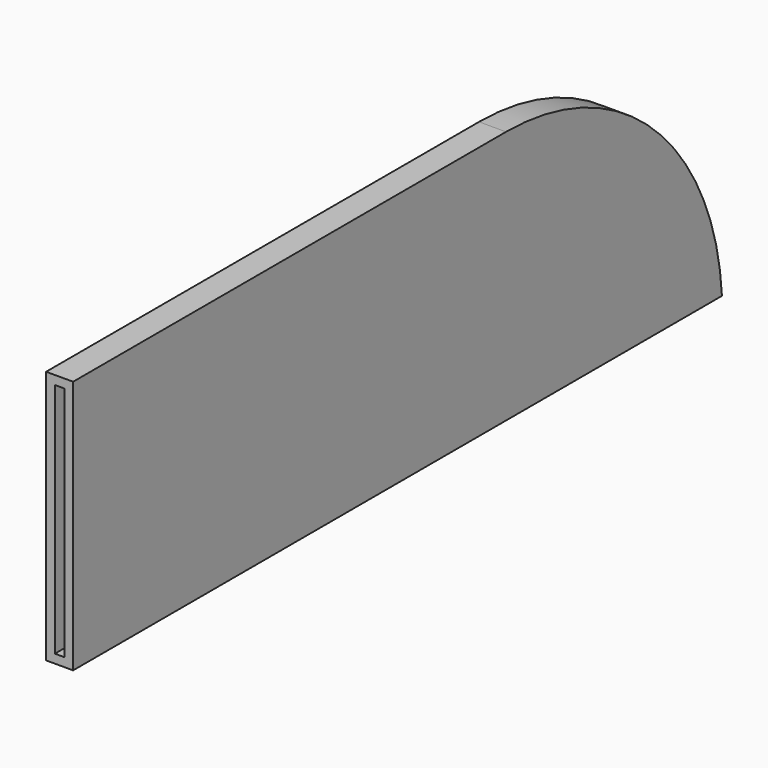
from build123d import *

# Parameters (mm, degrees)
F0_W        = 150
F0_H        = 47
F1_DEPTH    = 5
F2_T1_DEPTH = 254.5495942694
F3_T        = -1.625


# Not quite as in the source:
# - a fillet or chamfer that OpenCascade refuses, or shapes differently, is made with other operations: its cross-section is extruded or revolved along the edge and cut away or added


with BuildPart() as f1:
    # F0 (on Right) → F1 (new body)
    with BuildSketch(Plane.YZ):
        with Locations((9.6287353195, 42.6455706358)):
            Rectangle(F0_W, F0_H)
    extrude(amount=F1_DEPTH)

    # F2: fillet of radius 50 on 1 edges, made by hand

    # F2_s2 → F2_t1 (cut)
    with BuildSketch(Plane.YZ.offset(-124.7747971347)):
        with BuildLine():
            ThreePointArc((84.6287353195, 19.1455706358), (68.9970894677, 52.5461200822), (34.7188164657, 66.1455706358))
            Line((34.7188164657, 66.1455706358), (84.6287353195, 66.1455706358))
            Line((84.6287353195, 66.1455706358), (84.6287353195, 19.1455706358))
        make_face()
    extrude(amount=F2_T1_DEPTH, mode=Mode.SUBTRACT)

    # F3
    f3_openings = [f1.faces().sort_by_distance(p)[0] for p in [
        (2.5, -65.371265, 42.645571),
    ]]
    offset(amount=F3_T, openings=f3_openings)


solid = f1.part
